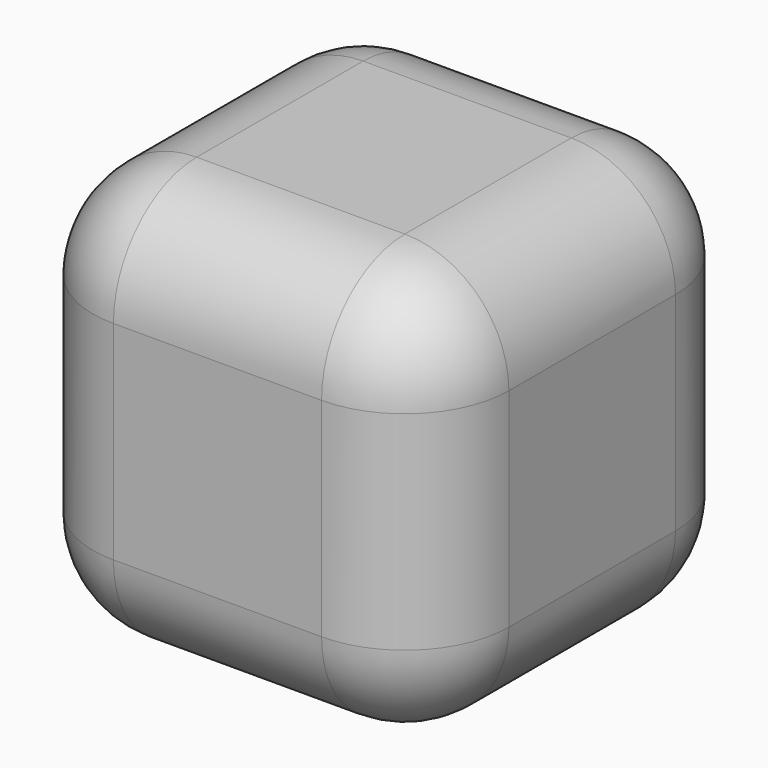
from build123d import *

# Parameters (mm, degrees)
F0_W         = 50.8
F0_H         = 50.8
F1_DEPTH     = 25.4
F2_DEPTH     = 25.4
F3_R         = 12.7
F4_R         = 12.7
F5_T1_DEPTH  = 25.4
F5_S5_W      = 12.7
F5_S5_H      = 12.7
F5_T6_DEPTH  = 12.7
F5_S11_W     = 12.7
F5_S11_H     = 12.7
F5_T12_DEPTH = 12.7
F5_S17_W     = 12.7
F5_S17_H     = 12.7
F5_T18_DEPTH = 12.7
F5_S23_W     = 12.7
F5_S23_H     = 12.7
F5_T24_DEPTH = 12.7
F5_S29_W     = 12.7
F5_S29_H     = 12.7
F5_T30_DEPTH = 12.7
F5_S35_W     = 12.7
F5_S35_H     = 12.7
F5_T36_DEPTH = 12.7
F5_S41_W     = 12.7
F5_S41_H     = 12.7
F5_T42_DEPTH = 12.7
F5_S47_W     = 12.7
F5_S47_H     = 12.7
F5_T48_DEPTH = 12.7


# Not quite as in the source:
# - a fillet or chamfer that OpenCascade refuses, or shapes differently, is made with other operations: its cross-section is extruded or revolved along the edge and cut away or added


with BuildPart() as f1:
    # F0 (on Top) → F1 (new body)
    with BuildSketch(Plane.XY):
        with Locations((-3.5267624348, -4.2439938247)):
            Rectangle(F0_W, F0_H)
    extrude(amount=F1_DEPTH)

    # F2 (add): a face of the model
    f2_faces = [f1.faces().sort_by_distance(p)[0] for p in [
        (-3.5267624348, -4.2439938247, 0),
    ]]
    extrude(f2_faces, amount=F2_DEPTH)

    # F3
    f3_edges = [f1.edges().sort_by_distance(p)[0] for p in [
        (-3.526762, -29.643994, 25.4),
        (-28.926762, -4.243994, 25.4),
        (-3.526762, 21.156006, 25.4),
        (21.873238, -4.243994, 25.4),
    ]]
    fillet(f3_edges, radius=F3_R)

    # F4
    f4_edges = [f1.edges().sort_by_distance(p)[0] for p in [
        (-3.526762, -29.643994, -25.4),
        (-28.926762, -4.243994, -25.4),
        (-3.526762, 21.156006, -25.4),
        (21.873238, -4.243994, -25.4),
    ]]
    fillet(f4_edges, radius=F4_R)

    # F5: fillet of radius 12.7 on 4 edges, made by hand

    # F5_s2 → F5_t1 (cut)
    with BuildSketch(Plane.XY.offset(-12.7)):
        with BuildLine():
            ThreePointArc((-28.9267624348, -16.9439938247), (-25.2070185559, -25.9242499458), (-16.2267624348, -29.6439938247))
            Line((-16.2267624348, -29.6439938247), (-28.9267624348, -29.6439938247))
            Line((-28.9267624348, -29.6439938247), (-28.9267624348, -16.9439938247))
        make_face()
        with BuildLine():
            ThreePointArc((-16.2267624348, 21.1560061753), (-25.2070185559, 17.4362622963), (-28.9267624348, 8.4560061753))
            Line((-28.9267624348, 8.4560061753), (-28.9267624348, 21.1560061753))
            Line((-28.9267624348, 21.1560061753), (-16.2267624348, 21.1560061753))
        make_face()
        with BuildLine():
            ThreePointArc((9.1732375652, 21.1560061753), (18.1534936862, 17.4362622963), (21.8732375652, 8.4560061753))
            Line((21.8732375652, 8.4560061753), (21.8732375652, 21.1560061753))
            Line((21.8732375652, 21.1560061753), (9.1732375652, 21.1560061753))
        make_face()
        with BuildLine():
            ThreePointArc((21.8732375652, -16.9439938247), (18.1534936862, -25.9242499458), (9.1732375652, -29.6439938247))
            Line((9.1732375652, -29.6439938247), (21.8732375652, -29.6439938247))
            Line((21.8732375652, -29.6439938247), (21.8732375652, -16.9439938247))
        make_face()
    extrude(amount=F5_T1_DEPTH, mode=Mode.SUBTRACT)


with BuildPart() as f5_tool4:
    # F5_s5 → F5_t6 (new body)
    with BuildSketch(Plane.YZ.offset(9.1732375652)):
        with Locations((-23.2939938247, 19.05)):
            Rectangle(F5_S5_W, F5_S5_H)
    extrude(amount=F5_T6_DEPTH)

    # F5_s7 → F5_t8 (revolve, cut)
    with BuildSketch(Plane(origin=(9.1732375652, -16.9439938247, 12.7), x_dir=(0, 0.7071067812, -0.7071067812), z_dir=(0, -0.7071067812, -0.7071067812))):
        with BuildLine():
            ThreePointArc((0, -12.7), (12.7, 0), (0, 12.7))
            Line((0, 12.7), (0, -12.7))
        make_face()
    revolve(axis=Axis((9.1732375652, -16.9439938247, 12.7), (1, 0, 0)), mode=Mode.SUBTRACT)


with BuildPart() as f1_1:
    add(f1.part)

    # F5_t3: cut F5_tool4
    add(f5_tool4.part, mode=Mode.SUBTRACT)


with BuildPart() as f5_tool10:
    # F5_s11 → F5_t12 (new body)
    with BuildSketch(Plane.YZ.offset(9.1732375652)):
        with Locations((-23.2939938247, -19.05)):
            Rectangle(F5_S11_W, F5_S11_H)
    extrude(amount=F5_T12_DEPTH)

    # F5_s13 → F5_t14 (revolve, cut)
    with BuildSketch(Plane(origin=(9.1732375652, -16.9439938247, -12.7), x_dir=(0, 0.7071067812, 0.7071067812), z_dir=(0, 0.7071067812, -0.7071067812))):
        with BuildLine():
            ThreePointArc((0, -12.7), (12.7, 0), (0, 12.7))
            Line((0, 12.7), (0, -12.7))
        make_face()
    revolve(axis=Axis((9.1732375652, -16.9439938247, -12.7), (1, 0, 0)), mode=Mode.SUBTRACT)


with BuildPart() as f1_2:
    add(f1_1.part)

    # F5_t9: cut F5_tool10
    add(f5_tool10.part, mode=Mode.SUBTRACT)


with BuildPart() as f5_tool16:
    # F5_s17 → F5_t18 (new body)
    with BuildSketch(Plane.XZ.offset(-8.4560061753)):
        with Locations((15.5232375652, 19.05)):
            Rectangle(F5_S17_W, F5_S17_H)
    extrude(amount=-F5_T18_DEPTH)

    # F5_s19 → F5_t20 (revolve, cut)
    with BuildSketch(Plane(origin=(9.1732375652, 8.4560061753, 12.7), x_dir=(-0.7071067812, 0, -0.7071067812), z_dir=(0.7071067812, 0, -0.7071067812))):
        with BuildLine():
            ThreePointArc((0, -12.7), (12.7, 0), (0, 12.7))
            Line((0, 12.7), (0, -12.7))
        make_face()
    revolve(axis=Axis((9.1732375652, 8.4560061753, 12.7), (0, 1, 0)), mode=Mode.SUBTRACT)


with BuildPart() as f1_3:
    add(f1_2.part)

    # F5_t15: cut F5_tool16
    add(f5_tool16.part, mode=Mode.SUBTRACT)


with BuildPart() as f5_tool22:
    # F5_s23 → F5_t24 (new body)
    with BuildSketch(Plane.XZ.offset(-8.4560061753)):
        with Locations((15.5232375652, -19.05)):
            Rectangle(F5_S23_W, F5_S23_H)
    extrude(amount=-F5_T24_DEPTH)

    # F5_s25 → F5_t26 (revolve, cut)
    with BuildSketch(Plane(origin=(9.1732375652, 8.4560061753, -12.7), x_dir=(-0.7071067812, 0, 0.7071067812), z_dir=(-0.7071067812, 0, -0.7071067812))):
        with BuildLine():
            ThreePointArc((0, -12.7), (12.7, 0), (0, 12.7))
            Line((0, 12.7), (0, -12.7))
        make_face()
    revolve(axis=Axis((9.1732375652, 8.4560061753, -12.7), (0, 1, 0)), mode=Mode.SUBTRACT)


with BuildPart() as f1_4:
    add(f1_3.part)

    # F5_t21: cut F5_tool22
    add(f5_tool22.part, mode=Mode.SUBTRACT)


with BuildPart() as f5_tool28:
    # F5_s29 → F5_t30 (new body)
    with BuildSketch(Plane.XZ.offset(-8.4560061753)):
        with Locations((-22.5767624348, -19.05)):
            Rectangle(F5_S29_W, F5_S29_H)
    extrude(amount=-F5_T30_DEPTH)

    # F5_s31 → F5_t32 (revolve, cut)
    with BuildSketch(Plane(origin=(-16.2267624348, 8.4560061753, -12.7), x_dir=(0.7071067812, 0, 0.7071067812), z_dir=(-0.7071067812, 0, 0.7071067812))):
        with BuildLine():
            ThreePointArc((0, -12.7), (12.7, 0), (0, 12.7))
            Line((0, 12.7), (0, -12.7))
        make_face()
    revolve(axis=Axis((-16.2267624348, 8.4560061753, -12.7), (0, 1, 0)), mode=Mode.SUBTRACT)


with BuildPart() as f1_5:
    add(f1_4.part)

    # F5_t27: cut F5_tool28
    add(f5_tool28.part, mode=Mode.SUBTRACT)


with BuildPart() as f5_tool34:
    # F5_s35 → F5_t36 (new body)
    with BuildSketch(Plane.XZ.offset(-8.4560061753)):
        with Locations((-22.5767624348, 19.05)):
            Rectangle(F5_S35_W, F5_S35_H)
    extrude(amount=-F5_T36_DEPTH)

    # F5_s37 → F5_t38 (revolve, cut)
    with BuildSketch(Plane(origin=(-16.2267624348, 8.4560061753, 12.7), x_dir=(0.7071067812, 0, -0.7071067812), z_dir=(0.7071067812, 0, 0.7071067812))):
        with BuildLine():
            ThreePointArc((0, -12.7), (12.7, 0), (0, 12.7))
            Line((0, 12.7), (0, -12.7))
        make_face()
    revolve(axis=Axis((-16.2267624348, 8.4560061753, 12.7), (0, 1, 0)), mode=Mode.SUBTRACT)


with BuildPart() as f1_6:
    add(f1_5.part)

    # F5_t33: cut F5_tool34
    add(f5_tool34.part, mode=Mode.SUBTRACT)


with BuildPart() as f5_tool40:
    # F5_s41 → F5_t42 (new body)
    with BuildSketch(Plane.YZ.offset(-16.2267624348)):
        with Locations((-23.2939938247, -19.05)):
            Rectangle(F5_S41_W, F5_S41_H)
    extrude(amount=-F5_T42_DEPTH)

    # F5_s43 → F5_t44 (revolve, cut)
    with BuildSketch(Plane(origin=(-16.2267624348, -16.9439938247, -12.7), x_dir=(0, 0.7071067812, 0.7071067812), z_dir=(0, -0.7071067812, 0.7071067812))):
        with BuildLine():
            ThreePointArc((0, -12.7), (12.7, 0), (0, 12.7))
            Line((0, 12.7), (0, -12.7))
        make_face()
    revolve(axis=Axis((-16.2267624348, -16.9439938247, -12.7), (-1, 0, 0)), mode=Mode.SUBTRACT)


with BuildPart() as f1_7:
    add(f1_6.part)

    # F5_t39: cut F5_tool40
    add(f5_tool40.part, mode=Mode.SUBTRACT)


with BuildPart() as f5_tool46:
    # F5_s47 → F5_t48 (new body)
    with BuildSketch(Plane.YZ.offset(-16.2267624348)):
        with Locations((-23.2939938247, 19.05)):
            Rectangle(F5_S47_W, F5_S47_H)
    extrude(amount=-F5_T48_DEPTH)

    # F5_s49 → F5_t50 (revolve, cut)
    with BuildSketch(Plane(origin=(-16.2267624348, -16.9439938247, 12.7), x_dir=(0, 0.7071067812, -0.7071067812), z_dir=(0, 0.7071067812, 0.7071067812))):
        with BuildLine():
            ThreePointArc((0, -12.7), (12.7, 0), (0, 12.7))
            Line((0, 12.7), (0, -12.7))
        make_face()
    revolve(axis=Axis((-16.2267624348, -16.9439938247, 12.7), (-1, 0, 0)), mode=Mode.SUBTRACT)


with BuildPart() as f1_8:
    add(f1_7.part)

    # F5_t45: cut F5_tool46
    add(f5_tool46.part, mode=Mode.SUBTRACT)


solid = f1_8.part
